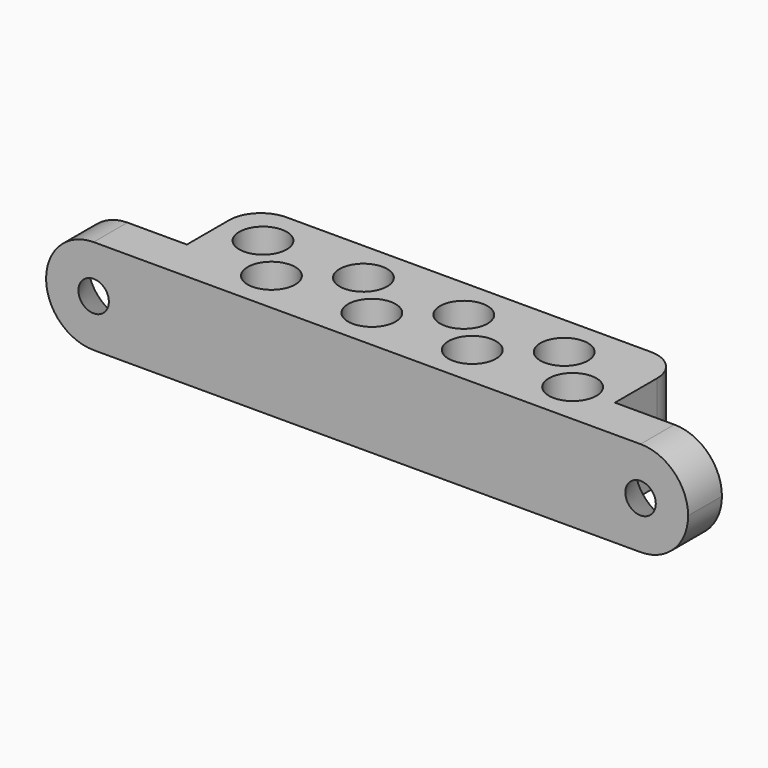
from build123d import *

# Parameters (mm, degrees)
F1_DEPTH = 3.81
F3_R     = 3.80999
F4_R     = 2.54
F2_R     = 1.905
F5_DEPTH = 3.81


# Not quite as in the source:
# - a fillet or chamfer is up to 0.001 mm smaller than in the source, because OpenCascade refuses the exact size
# - a pattern or mirror of a feature is missing from the dataset's text; its kind, count and spacing are read off the source's solid


with BuildPart() as f1:
    # F0 (on Top) → F1 (new body, symmetric)
    with BuildSketch(Plane.XY):
        Polygon((17.145, 10.16), (0, 10.16), (-17.145, 10.16), (-17.145, 3.38582), (-25.7175, 3.38582), (-25.7175, 0), (0, 0), (25.7175, 0), (25.7175, 3.38582), (17.145, 3.38582), align=None)
    extrude(amount=F1_DEPTH, both=True)

    # F3 (radius 3.81 in the source; OpenCascade refuses exactly that, so slightly less here)
    f3_edges = [f1.edges().sort_by_distance(p)[0] for p in [
        (-25.7175, 1.69291, 3.81),
        (-25.7175, 1.69291, -3.81),
        (25.7175, 1.69291, 3.81),
        (25.7175, 1.69291, -3.81),
    ]]
    fillet(f3_edges, radius=F3_R)

    # F4
    f4_edges = [f1.edges().sort_by_distance(p)[0] for p in [
        (-17.145, 10.16, 0),
        (17.145, 10.16, 0),
    ]]
    fillet(f4_edges, radius=F4_R)

    # F2 (on Top) → F5 (cut, symmetric)
    with BuildSketch(Plane.XY):
        with Locations((-13.7583333333, 6.7733333333)):
            Circle(F2_R)
        with Locations((-10.3716666667, 3.3866666667)):
            Circle(F2_R)
        with Locations((-2.3283333333, 3.3866666667)):
            Circle(F2_R)
        with Locations((-5.715, 6.7733333333)):
            Circle(F2_R)
        with Locations((5.715, 3.3866666667)):
            Circle(F2_R)
        with Locations((2.3283333333, 6.7733333333)):
            Circle(F2_R)
        with Locations((13.7583333333, 3.3866666667)):
            Circle(F2_R)
        with Locations((10.3716666667, 6.7733333333)):
            Circle(F2_R)
    extrude(amount=F5_DEPTH, both=True, mode=Mode.SUBTRACT)

    # F6 (on Top) → F7 (revolve, cut)
    with BuildSketch(Plane.XY):
        Polygon((-21.9075, -2.113441314), (-21.9075, 3.38582), (-25.0825, 3.38582), align=None)
    f7 = revolve(axis=Axis((-21.9075, 0.636189343, 0), (0, 1, 0)), mode=Mode.SUBTRACT)

    # F7_copies: F7 across plane
    add(f7.mirror(Plane(origin=(0, 0, 0), x_dir=(0, 0, 1), z_dir=(1, 0, 0))), mode=Mode.SUBTRACT)


solid = f1.part
